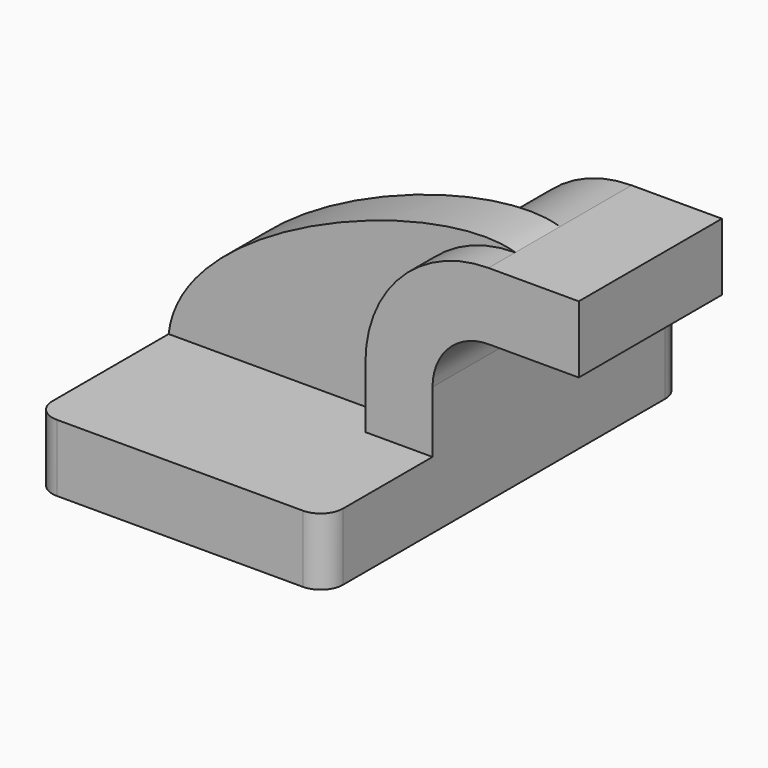
from build123d import *

# Parameters (mm, degrees)
F1_DEPTH = 63.5
F0_W     = 22.4716843884
F0_H     = 19.05
F2_DEPTH = 25.4
F3_DEPTH = 15.875
F5_R     = 6.35


# Not quite as in the source:
# - the program builds the solid bodies; features that only make, move or delete a surface that nothing else refers to are left out


with BuildPart() as f1:
    # F0 (on Front) → F1 (new body, symmetric)
    with BuildSketch(Plane.XZ):
        Polygon((22.225, 9.525), (-41.275, 9.525), (-41.275, -9.525), (41.275, -9.525), (41.275, 9.525), align=None)
    extrude(amount=F1_DEPTH, both=True)

    # F0 (on Front) → F2 (join, symmetric)
    with BuildSketch(Plane.XZ):
        with BuildLine():
            Line((22.225, 27.0002), (22.225, 9.525))
            Line((22.225, 9.525), (41.275, 9.525))
            Line((41.275, 9.525), (41.275, 27.0002))
            ThreePointArc((41.275, 27.0002), (45.9246798487, 38.2255201513), (57.15, 42.8752))
            Line((57.15, 42.8752), (60.325, 42.8752))
            Line((60.325, 42.8752), (60.325, 61.9252))
            Line((60.325, 61.9252), (57.15, 61.9252))
            ThreePointArc((57.15, 61.9252), (32.4542956671, 51.6959043329), (22.225, 27.0002))
        make_face()
        with Locations((71.5608421942, 52.4002)):
            Rectangle(F0_W, F0_H)
    extrude(amount=F2_DEPTH, both=True)

    # F0 (on Front) → F3 (join)
    with BuildSketch(Plane.XZ):
        with BuildLine():
            add(Edge.make_bspline(
                [(-41.275, 9.525), (-37.7052687109, 41.8739132583), (35.1902469993, 68.9807906747), (57.15, 61.9252)],
                knots=[0, 0, 0, 0, 111.5045361635, 111.5045361635, 111.5045361635, 111.5045361635], degree=3))
            Line((-41.275, 9.525), (22.225, 9.525))
            Line((22.225, 9.525), (22.225, 27.0002))
            ThreePointArc((22.225, 27.0002), (32.4542956671, 51.6959043329), (57.15, 61.9252))
        make_face()
    extrude(amount=F3_DEPTH)

    # F5
    f5_edges = [f1.edges().sort_by_distance(p)[0] for p in [
        (41.275, -63.5, 0),
        (-41.275, -63.5, 0),
        (-41.275, 63.5, 0),
        (41.275, 63.5, 0),
    ]]
    fillet(f5_edges, radius=F5_R)


solid = f1.part
